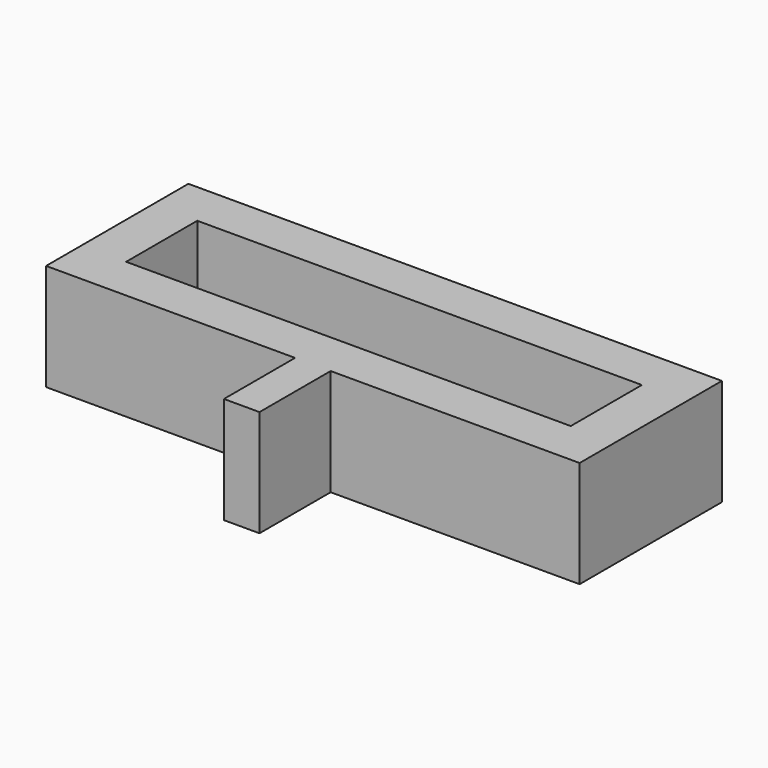
from build123d import *

# Parameters (mm, degrees)
F0_W        = 2
F0_H        = 5
F1_DEPTH    = 6
F2_T        = 2.5
F2_T3_DEPTH = 11


# Not quite as in the source:
# - a shell that OpenCascade refuses in one call is made with other operations: the cavity is built on its own and cut out


with BuildPart() as f1:
    # F0 (on Top) → F1 (new body)
    with BuildSketch(Plane.XY):
        Polygon((30, 0), (0, 0), (0, -10), (14, -10), (14, -5), (16, -5), (16, -10), (30, -10), align=None)
        with Locations((15, -7.5)):
            Rectangle(F0_W, F0_H)
        with Locations((15, -12.5)):
            Rectangle(F0_W, F0_H)
    extrude(amount=F1_DEPTH)

    # F2: shell of thickness 2.5, made by hand


with BuildPart() as f2_core1:
    # F2_t2: copy of F1
    add(f1.part)

    # the walls: a layer under each face that stays
    f2_faces = [f2_core1.faces().sort_by_distance(p)[0] for p in [
        (15, 0, 3),
        (0, -5, 3),
        (7, -10, 3),
        (14, -12.5, 3),
        (15, -15, 3),
        (16, -12.5, 3),
        (23, -10, 3),
        (30, -5, 3),
        (15, -7.5, 0),
    ]]
    thicken(f2_faces, amount=-F2_T, mode=Mode.SUBTRACT)

    # F2_s4 → F2_t3 (cut)
    with BuildSketch(Plane.XY.offset(-2.5)):
        Polygon((13.975, -10.025), (14, -7.5), (16.5, -7.5), (16.5, -10), align=None)
        Polygon((16.025, -10.025), (13.5, -10), (13.5, -7.5), (16, -7.5), align=None)
    extrude(amount=F2_T3_DEPTH, mode=Mode.SUBTRACT)


with BuildPart() as f1_1:
    add(f1.part)

    # what is left inside the walls is the cavity
    f2_cavity = [f2_core1.part.solids().sort_by_distance(p)[0] for p in [
        (15, -5.833333, 5.975),
    ]]
    add(f2_cavity, mode=Mode.SUBTRACT)


solid = f1_1.part
